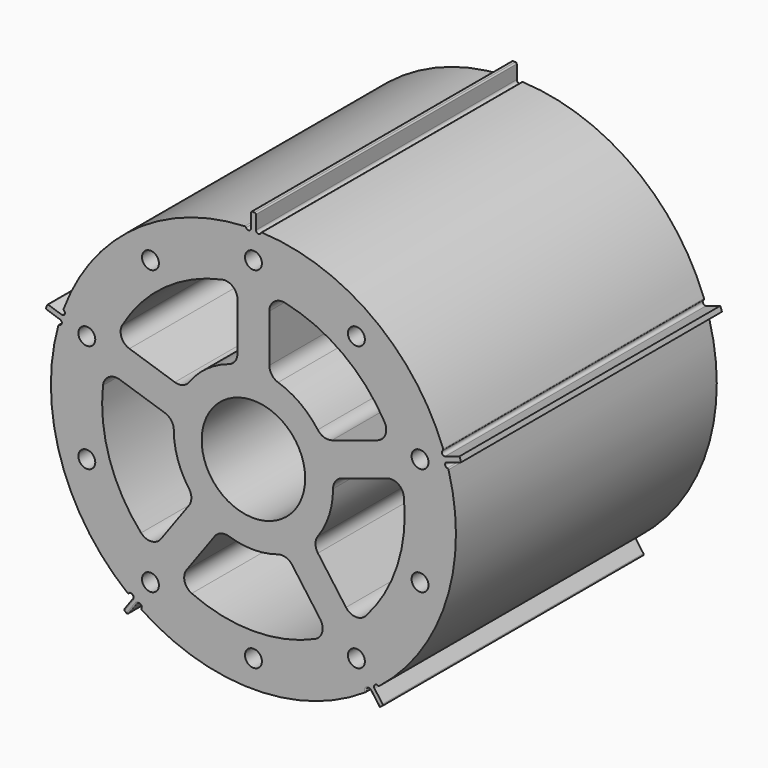
from build123d import *

# Parameters (mm, degrees)
F1_DEPTH = 129.9972
F2_R     = 20.6375
F3_DEPTH = 129.9972
F5_R     = 1.016
F6_DEPTH = 129.9982
F7_R     = 0.508
F9_DEPTH = 129.9982001
F10_R    = 5.08
F12_D    = 6.7564


with BuildPart() as f1:
    # F0 (on Front) → F1 (new body)
    with BuildSketch(Plane.XZ):
        with BuildLine():
            Line((-1.000252, 86.7377727848), (-1.000252, 80.7429446248))
            ThreePointArc((-1.000252, 80.7429446248), (-47.4631536273, 65.3274265412), (-76.4820087636, 25.9022382475))
            Line((-76.4820087636, 25.9022382475), (-82.1834291493, 27.7547420273))
            Line((-82.1834291493, 27.7547420273), (-82.8016188826, 25.8521496622))
            Line((-82.8016188826, 25.8521496622), (-77.1001984969, 23.9996458824))
            ThreePointArc((-77.1001984969, 23.9996458824), (-76.7969957822, -24.9528565412), (-48.2687329438, -64.7344810031))
            Line((-48.2687329438, -64.7344810031), (-51.7924045263, -69.584398863))
            Line((-51.7924045263, -69.584398863), (-50.1739627929, -70.7602656113))
            Line((-50.1739627929, -70.7602656113), (-46.6502912104, -65.9103477515))
            ThreePointArc((-46.6502912104, -65.9103477515), (0, -80.74914), (46.6502912104, -65.9103477515))
            ThreePointArc((46.6502912104, -65.9103477515), (47.4631536273, -65.3274265412), (48.2687329438, -64.7344810031))
            ThreePointArc((48.2687329438, -64.7344810031), (76.7969957822, -24.9528565412), (77.1001984969, 23.9996458824))
            Line((77.1001984969, 23.9996458824), (82.8016188826, 25.8521496622))
            Line((82.8016188826, 25.8521496622), (82.1834291493, 27.7547420273))
            Line((82.1834291493, 27.7547420273), (76.4820087636, 25.9022382475))
            ThreePointArc((76.4820087636, 25.9022382475), (47.4631536273, 65.3274265412), (1.000252, 80.7429446248))
            Line((1.000252, 80.7429446248), (1.000252, 86.7377727848))
            Line((1.000252, 86.7377727848), (-1.000252, 86.7377727848))
        make_face()
        with BuildLine():
            Line((51.7924045263, -69.584398863), (48.2687329438, -64.7344810031))
            ThreePointArc((48.2687329438, -64.7344810031), (47.4631536273, -65.3274265412), (46.6502912104, -65.9103477515))
            Line((46.6502912104, -65.9103477515), (50.1739627929, -70.7602656113))
            Line((50.1739627929, -70.7602656113), (51.7924045263, -69.584398863))
        make_face()
    extrude(amount=F1_DEPTH)

    # F2 (on Front) → F3 (cut, through all)
    with BuildSketch(Plane.XZ):
        Circle(F2_R)
    extrude(amount=F3_DEPTH, mode=Mode.SUBTRACT)

    # F5 (on face) → F6 (cut, through all)
    with BuildSketch(Plane(origin=(0, 0, 0), x_dir=(-1, 0, 0), z_dir=(0, 1, 0))):
        with Locations((-2.016252, 80.7429446248)):
            Circle(F5_R)
        with Locations((2.016252, 80.7429446248)):
            Circle(F5_R)
        with Locations((-76.1680474973, 26.868511668)):
            Circle(F5_R)
        with Locations((-77.4141597632, 23.0333724618)):
            Circle(F5_R)
        with Locations((-49.09069421, -64.1372911868)):
            Circle(F5_R)
        with Locations((-45.8283299442, -66.5075375678)):
            Circle(F5_R)
        with Locations((45.8283299442, -66.5075375678)):
            Circle(F5_R)
        with Locations((49.09069421, -64.1372911868)):
            Circle(F5_R)
        with Locations((77.4141597632, 23.0333724618)):
            Circle(F5_R)
        with Locations((76.1680474973, 26.868511668)):
            Circle(F5_R)
    extrude(amount=-F6_DEPTH, mode=Mode.SUBTRACT)

    # F7
    f7_edges = [f1.edges().sort_by_distance(p)[0] for p in [
        (-1.000252, -64.9986, 86.737773),
        (1.000252, -64.9986, 86.737773),
        (-3.030986, -64.9986, 80.692235),
        (3.030986, -64.9986, 80.692235),
        (-82.183429, -64.9986, 27.754742),
        (-82.801619, -64.9986, 25.85215),
        (-51.792405, -64.9986, -69.584399),
        (-50.173963, -64.9986, -70.760266),
        (49.881824, -64.9986, -63.49982),
        (77.679502, -64.9986, 22.052633),
        (50.173963, -64.9986, -70.760266),
        (51.792405, -64.9986, -69.584399),
        (75.80625, -64.9986, 27.817911),
        (-48.473171, -129.9972, -63.330494),
        (-50.030569, -129.9972, -67.15944),
        (-48.412127, -129.9972, -68.335307),
        (-45.251845, -129.9972, -65.670925),
        (45.251845, -129.9972, -65.670925),
        (48.412127, -129.9972, -68.335307),
        (44.977587, -64.9986, -67.062958),
        (-44.977587, -64.9986, -67.062958),
        (-49.881824, -64.9986, -63.49982),
        (-77.679502, -64.9986, 22.052633),
        (-75.80625, -64.9986, 27.817911),
    ]]
    fillet(f7_edges, radius=F7_R)

    # F8 (on face) → F9 (cut, through all)
    with BuildSketch(Plane(origin=(0, 0, 0), x_dir=(-1, 0, 0), z_dir=(0, 1, 0))):
        with BuildLine():
            Line((-6.35, 31.1085197333), (-6.35, 59.9898585179))
            ThreePointArc((-6.35, 59.9898585179), (-35.4581453445, 48.8039501857), (-55.0914879408, 24.5770946507))
            Line((-55.0914879408, 24.5770946507), (-27.6237024904, 15.6522701459))
            ThreePointArc((-27.6237024904, 15.6522701459), (-18.6621817603, 25.6862895714), (-6.35, 31.1085197333))
        make_face()
        with BuildLine():
            ThreePointArc((55.0914879408, 24.5770946507), (35.4581453445, 48.8039501857), (6.35, 59.9898585179))
            Line((6.35, 59.9898585179), (6.35, 31.1085197333))
            ThreePointArc((6.35, 31.1085197333), (18.6621817603, 25.6862895714), (27.6237024904, 15.6522701459))
            Line((27.6237024904, 15.6522701459), (55.0914879408, 24.5770946507))
        make_face()
        with BuildLine():
            Line((23.4223870342, -21.4348847821), (40.3984120382, -44.8003786791))
            ThreePointArc((40.3984120382, -44.8003786791), (57.3724843455, -18.6414501857), (59.0160037694, 12.4986768937))
            Line((59.0160037694, 12.4986768937), (31.548218319, 3.573852389))
            ThreePointArc((31.548218319, 3.573852389), (30.1960443924, -9.8112895714), (23.4223870342, -21.4348847821))
        make_face()
        with BuildLine():
            Line((-13.1478712056, -28.8997574862), (-30.1238962097, -52.2652513832))
            ThreePointArc((-30.1238962097, -52.2652513832), (0, -60.325), (30.1238962097, -52.2652513832))
            Line((30.1238962097, -52.2652513832), (13.1478712056, -28.8997574862))
            ThreePointArc((13.1478712056, -28.8997574862), (0, -31.75), (-13.1478712056, -28.8997574862))
        make_face()
        with BuildLine():
            Line((-31.548218319, 3.573852389), (-59.0160037694, 12.4986768937))
            ThreePointArc((-59.0160037694, 12.4986768937), (-57.3724843455, -18.6414501857), (-40.3984120382, -44.8003786791))
            Line((-40.3984120382, -44.8003786791), (-23.4223870342, -21.4348847821))
            ThreePointArc((-23.4223870342, -21.4348847821), (-30.1960443924, -9.8112895714), (-31.548218319, 3.573852389))
        make_face()
    extrude(amount=-F9_DEPTH, mode=Mode.SUBTRACT)

    # F10
    f10_edges = [f1.edges().sort_by_distance(p)[0] for p in [
        (55.091488, -64.9986, 24.577095),
        (27.623702, -64.9986, 15.65227),
        (6.35, -64.9986, 31.10852),
        (6.35, -64.9986, 59.989859),
        (-55.091488, -64.9986, 24.577095),
        (-27.623702, -64.9986, 15.65227),
        (-6.35, -64.9986, 31.10852),
        (-6.35, -64.9986, 59.989859),
        (-59.016004, -64.9986, 12.498677),
        (-40.398412, -64.9986, -44.800379),
        (-23.422387, -64.9986, -21.434885),
        (-31.548218, -64.9986, 3.573852),
        (30.123896, -64.9986, -52.265251),
        (-30.123896, -64.9986, -52.265251),
        (-13.147871, -64.9986, -28.899757),
        (13.147871, -64.9986, -28.899757),
        (31.548218, -64.9986, 3.573852),
        (23.422387, -64.9986, -21.434885),
        (40.398412, -64.9986, -44.800379),
        (59.016004, -64.9986, 12.498677),
    ]]
    fillet(f10_edges, radius=F10_R)

    # F12 (through all)
    with Locations(Plane(origin=(0, 0, 0), x_dir=(-1, 0, 0), z_dir=(0, 1, 0))):
        with Locations((0, 69.85), (-41.0567998726, 56.5098370571), (-66.4312976632, 21.5848370571), (-66.4312976632, -21.5848370571), (-41.0567998726, -56.5098370571), (0, -69.85), (41.0567998726, -56.5098370571), (66.4312976632, -21.5848370571), (66.4312976632, 21.5848370571), (41.0567998726, 56.5098370571)):
            Hole(F12_D / 2)


solid = f1.part
